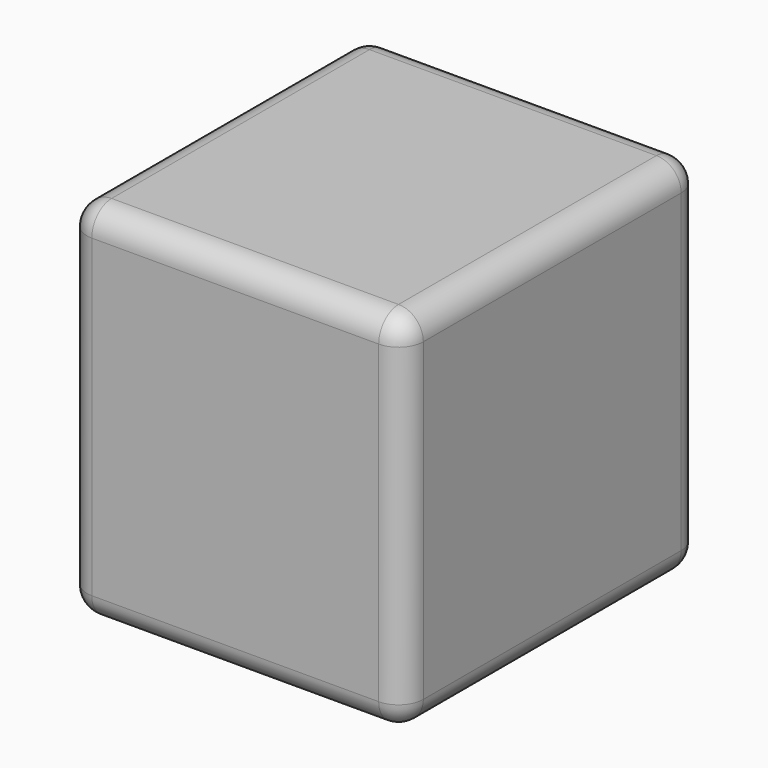
from build123d import *

# Parameters (mm, degrees)
F0_W         = 68.9483396709
F0_H         = 74.6622905135
F1_DEPTH     = 76.2
F2_R         = 5.08
F3_R         = 5.08
F4_R         = 5.08
F5_T1_DEPTH  = 66.04
F5_T3_DEPTH  = 58.7883396709
F5_S7_W      = 5.08
F5_S7_H      = 5.08
F5_T8_DEPTH  = 5.08
F5_S13_W     = 5.08
F5_S13_H     = 5.08
F5_T14_DEPTH = 5.08
F5_T18_ANGLE = 90
F5_T20_ANGLE = 90
F6_T1_DEPTH  = 58.7883396709
F6_T3_DEPTH  = 66.04
F6_S7_W      = 5.08
F6_S7_H      = 5.08
F6_T8_DEPTH  = 5.08
F6_S13_W     = 5.08
F6_S13_H     = 5.08
F6_T14_DEPTH = 5.08
F6_T18_ANGLE = 90
F6_T20_ANGLE = 90


# Not quite as in the source:
# - a fillet or chamfer that OpenCascade refuses, or shapes differently, is made with other operations: its cross-section is extruded or revolved along the edge and cut away or added


with BuildPart() as f1:
    # F0 (on Front) → F1 (new body)
    with BuildSketch(Plane.XZ):
        with Locations((0.3492366523, -0.4755854607)):
            Rectangle(F0_W, F0_H)
    extrude(amount=F1_DEPTH)

    # F2
    f2_edges = [f1.edges().sort_by_distance(p)[0] for p in [
        (34.823406, -76.2, -0.475585),
        (0.349237, -76.2, 36.85556),
        (-34.124933, -76.2, -0.475585),
        (0.349237, -76.2, -37.806731),
    ]]
    fillet(f2_edges, radius=F2_R)

    # F3
    f3_edges = [f1.edges().sort_by_distance(p)[0] for p in [
        (34.823406, 0, -0.475585),
    ]]
    fillet(f3_edges, radius=F3_R)

    # F4
    f4_edges = [f1.edges().sort_by_distance(p)[0] for p in [
        (-34.124933, 0, -0.475585),
    ]]
    fillet(f4_edges, radius=F4_R)

    # F5: fillet of radius 5.08 on 1 edges, made by hand

    # F5_s2 → F5_t1 (cut)
    with BuildSketch(Plane.XZ.offset(5.08)):
        with BuildLine():
            ThreePointArc((34.8234064877, 31.7755597961), (33.3355089361, 35.3676622445), (29.7434064877, 36.8555597961))
            Line((29.7434064877, 36.8555597961), (34.8234064877, 36.8555597961))
            Line((34.8234064877, 36.8555597961), (34.8234064877, 31.7755597961))
        make_face()
        with BuildLine():
            ThreePointArc((-34.1249331832, 31.7755597961), (-32.6370356316, 35.3676622445), (-29.0449331832, 36.8555597961))
            Line((-29.0449331832, 36.8555597961), (-34.1249331832, 36.8555597961))
            Line((-34.1249331832, 36.8555597961), (-34.1249331832, 31.7755597961))
        make_face()
    extrude(amount=F5_T1_DEPTH, mode=Mode.SUBTRACT)

    # F5_s4 → F5_t3 (cut)
    with BuildSketch(Plane.YZ.offset(-29.0449331832)):
        with BuildLine():
            ThreePointArc((0, 31.7755597961), (-1.4878975516, 35.3676622445), (-5.08, 36.8555597961))
            Line((-5.08, 36.8555597961), (0, 36.8555597961))
            Line((0, 36.8555597961), (0, 31.7755597961))
        make_face()
    extrude(amount=F5_T3_DEPTH, mode=Mode.SUBTRACT)


with BuildPart() as f5_tool6:
    # F5_s7 → F5_t8 (new body)
    with BuildSketch(Plane.YZ.offset(29.7434064877)):
        with Locations((-73.66, 34.3155597961)):
            Rectangle(F5_S7_W, F5_S7_H)
    extrude(amount=F5_T8_DEPTH)

    # F5_s9 → F5_t10 (revolve, cut)
    with BuildSketch(Plane(origin=(29.7434064877, -71.12, 31.7755597961), x_dir=(0, 0.7071067812, -0.7071067812), z_dir=(0, -0.7071067812, -0.7071067812))):
        with BuildLine():
            ThreePointArc((0, -5.08), (5.08, 0), (0, 5.08))
            Line((0, 5.08), (0, -5.08))
        make_face()
    revolve(axis=Axis((29.7434064877, -71.12, 31.7755597961), (1, 0, 0)), mode=Mode.SUBTRACT)


with BuildPart() as f1_1:
    add(f1.part)

    # F5_t5: cut F5_tool6
    add(f5_tool6.part, mode=Mode.SUBTRACT)


with BuildPart() as f5_tool12:
    # F5_s13 → F5_t14 (new body)
    with BuildSketch(Plane.YZ.offset(-29.0449331832)):
        with Locations((-73.66, 34.3155597961)):
            Rectangle(F5_S13_W, F5_S13_H)
    extrude(amount=-F5_T14_DEPTH)

    # F5_s15 → F5_t16 (revolve, cut)
    with BuildSketch(Plane(origin=(-29.0449331832, -71.12, 31.7755597961), x_dir=(0, 0.7071067812, -0.7071067812), z_dir=(0, 0.7071067812, 0.7071067812))):
        with BuildLine():
            ThreePointArc((0, -5.08), (5.08, 0), (0, 5.08))
            Line((0, 5.08), (0, -5.08))
        make_face()
    revolve(axis=Axis((-29.0449331832, -71.12, 31.7755597961), (-1, 0, 0)), mode=Mode.SUBTRACT)


with BuildPart() as f1_2:
    add(f1_1.part)

    # F5_t11: cut F5_tool12
    add(f5_tool12.part, mode=Mode.SUBTRACT)

    # F5_s17 → F5_t18 (revolve, cut)
    with BuildSketch(Plane.XZ.offset(5.08)):
        with BuildLine():
            ThreePointArc((34.8234064877, 31.7755597961), (33.3355089361, 35.3676622445), (29.7434064877, 36.8555597961))
            Line((29.7434064877, 36.8555597961), (34.8234064877, 36.8555597961))
            Line((34.8234064877, 36.8555597961), (34.8234064877, 31.7755597961))
        make_face()
    revolve(axis=Axis((29.7434064877, -5.08, 36.8555597961), (0, 0, 1)), revolution_arc=F5_T18_ANGLE, mode=Mode.SUBTRACT)

    # F5_s19 → F5_t20 (revolve, cut)
    with BuildSketch(Plane.YZ.offset(-29.0449331832)):
        with BuildLine():
            ThreePointArc((0, 31.7755597961), (-1.4878975516, 35.3676622445), (-5.08, 36.8555597961))
            Line((-5.08, 36.8555597961), (0, 36.8555597961))
            Line((0, 36.8555597961), (0, 31.7755597961))
        make_face()
    revolve(axis=Axis((-29.0449331832, -5.08, 36.8555597961), (0, 0, 1)), revolution_arc=F5_T20_ANGLE, mode=Mode.SUBTRACT)

    # F6: fillet of radius 5.08 on 1 edges, made by hand

    # F6_s2 → F6_t1 (cut)
    with BuildSketch(Plane.YZ.offset(-29.0449331832)):
        with BuildLine():
            ThreePointArc((-5.08, -37.8067307174), (-1.4878975516, -36.3188331658), (0, -32.7267307174))
            Line((0, -32.7267307174), (0, -37.8067307174))
            Line((0, -37.8067307174), (-5.08, -37.8067307174))
        make_face()
    extrude(amount=F6_T1_DEPTH, mode=Mode.SUBTRACT)

    # F6_s4 → F6_t3 (cut)
    with BuildSketch(Plane.XZ.offset(5.08)):
        with BuildLine():
            ThreePointArc((29.7434064877, -37.8067307174), (33.3355089361, -36.3188331658), (34.8234064877, -32.7267307174))
            Line((34.8234064877, -32.7267307174), (34.8234064877, -37.8067307174))
            Line((34.8234064877, -37.8067307174), (29.7434064877, -37.8067307174))
        make_face()
        with BuildLine():
            ThreePointArc((-29.0449331832, -37.8067307174), (-32.6370356316, -36.3188331658), (-34.1249331832, -32.7267307174))
            Line((-34.1249331832, -32.7267307174), (-34.1249331832, -37.8067307174))
            Line((-34.1249331832, -37.8067307174), (-29.0449331832, -37.8067307174))
        make_face()
    extrude(amount=F6_T3_DEPTH, mode=Mode.SUBTRACT)


with BuildPart() as f6_tool6:
    # F6_s7 → F6_t8 (new body)
    with BuildSketch(Plane.XY.offset(-32.7267307174)):
        with Locations((32.2834064877, -73.66)):
            Rectangle(F6_S7_W, F6_S7_H)
    extrude(amount=-F6_T8_DEPTH)

    # F6_s9 → F6_t10 (revolve, cut)
    with BuildSketch(Plane(origin=(29.7434064877, -71.12, -32.7267307174), x_dir=(-0.7071067812, 0.7071067812, 0), z_dir=(-0.7071067812, -0.7071067812, 0))):
        with BuildLine():
            ThreePointArc((0, -5.08), (5.08, 0), (0, 5.08))
            Line((0, 5.08), (0, -5.08))
        make_face()
    revolve(axis=Axis((29.7434064877, -71.12, -32.7267307174), (0, 0, -1)), mode=Mode.SUBTRACT)


with BuildPart() as f1_3:
    add(f1_2.part)

    # F6_t5: cut F6_tool6
    add(f6_tool6.part, mode=Mode.SUBTRACT)


with BuildPart() as f6_tool12:
    # F6_s13 → F6_t14 (new body)
    with BuildSketch(Plane.XY.offset(-32.7267307174)):
        with Locations((-31.5849331832, -73.66)):
            Rectangle(F6_S13_W, F6_S13_H)
    extrude(amount=-F6_T14_DEPTH)

    # F6_s15 → F6_t16 (revolve, cut)
    with BuildSketch(Plane(origin=(-29.0449331832, -71.12, -32.7267307174), x_dir=(0.7071067812, 0.7071067812, 0), z_dir=(-0.7071067812, 0.7071067812, 0))):
        with BuildLine():
            ThreePointArc((0, -5.08), (5.08, 0), (0, 5.08))
            Line((0, 5.08), (0, -5.08))
        make_face()
    revolve(axis=Axis((-29.0449331832, -71.12, -32.7267307174), (0, 0, -1)), mode=Mode.SUBTRACT)


with BuildPart() as f1_4:
    add(f1_3.part)

    # F6_t11: cut F6_tool12
    add(f6_tool12.part, mode=Mode.SUBTRACT)

    # F6_s17 → F6_t18 (revolve, cut)
    with BuildSketch(Plane.YZ.offset(-29.0449331832)):
        with BuildLine():
            ThreePointArc((-5.08, -37.8067307174), (-1.4878975516, -36.3188331658), (0, -32.7267307174))
            Line((0, -32.7267307174), (0, -37.8067307174))
            Line((0, -37.8067307174), (-5.08, -37.8067307174))
        make_face()
    revolve(axis=Axis((-29.0449331832, -5.08, -37.8067307174), (0, 0, 1)), revolution_arc=F6_T18_ANGLE, mode=Mode.SUBTRACT)

    # F6_s19 → F6_t20 (revolve, cut)
    with BuildSketch(Plane.XZ.offset(5.08)):
        with BuildLine():
            ThreePointArc((29.7434064877, -37.8067307174), (33.3355089361, -36.3188331658), (34.8234064877, -32.7267307174))
            Line((34.8234064877, -32.7267307174), (34.8234064877, -37.8067307174))
            Line((34.8234064877, -37.8067307174), (29.7434064877, -37.8067307174))
        make_face()
    revolve(axis=Axis((29.7434064877, -5.08, -37.8067307174), (0, 0, 1)), revolution_arc=F6_T20_ANGLE, mode=Mode.SUBTRACT)


solid = f1_4.part
